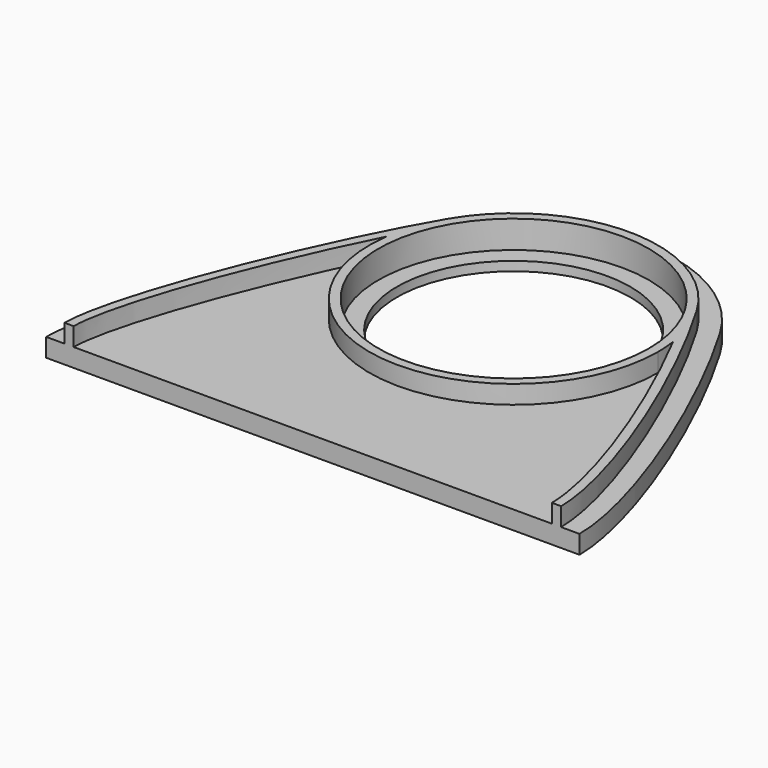
from build123d import *

# Parameters (mm, degrees)
F0_R     = 12.7
F1_DEPTH = 2
F3_DEPTH = 2
F4_DEPTH = 1


# Not quite as in the source:
# - the dataset's text gives a spline's control points without its knots; the knots are read off the source's solid


with BuildPart() as f1:
    # F0 (on Top) → F1 (new body)
    with BuildSketch(Plane.XY):
        with BuildLine():
            add(Edge.make_bspline(
                [(15.2512199078, 66.2827774838), (22.262781729, 54.3783446484), (29, 37.1850712509), (29, 30)],
                knots=[0, 0, 0, 0, 38.8003723689, 38.8003723689, 38.8003723689, 38.8003723689], degree=3))
            ThreePointArc((15.2512199078, 66.2827774838), (0, 75), (-15.2512199078, 66.2827774838))
            add(Edge.make_bspline(
                [(-15.2512199078, 66.2827774838), (-21.2251645455, 56.1400411697), (-29, 37.1850712509), (-29, 30)],
                knots=[0, 0, 0, 0, 38.8003723689, 38.8003723689, 38.8003723689, 38.8003723689], degree=3))
            Line((-29, 30), (-27, 30))
            Line((-27, 30), (27, 30))
            Line((27, 30), (29, 30))
        make_face()
        with Locations((0, 57.3)):
            Circle(F0_R, mode=Mode.SUBTRACT)
    extrude(amount=F1_DEPTH)

    # F2 (on face) → F3 (join)
    with BuildSketch(Plane.XY.offset(2)):
        with BuildLine():
            ThreePointArc((15.5364060101, 59.5605504394), (14.8096872708, 62.5118291359), (13.5279182233, 65.2677743783))
            ThreePointArc((13.5279182233, 65.2677743783), (0, 73), (-13.5279182233, 65.2677743783))
            ThreePointArc((-13.5279182233, 65.2677743783), (-14.8291754406, 62.4561182834), (-15.5529629237, 59.4436754174))
            add(Edge.make_bspline(
                [(-12.666267381, 64.7602728256), (-13.3814975344, 63.5459343458), (-14.3471757573, 61.795170814), (-15.3337673015, 59.8762099433), (-15.5529629237, 59.4436754174)],
                knots=[0, 0, 0, 0, 0.125, 0.160588695, 0.160588695, 0.160588695, 0.160588695], degree=3))
            ThreePointArc((-12.666267381, 64.7602728256), (0, 72), (12.666267381, 64.7602728256))
            add(Edge.make_bspline(
                [(12.666267381, 64.7602728256), (13.6300436519, 63.1239455453), (14.5936812112, 61.3751520533), (15.5364060101, 59.5605504394)],
                knots=[0, 0, 0, 0, 0.1417988525, 0.1417988525, 0.1417988525, 0.1417988525], degree=3))
        make_face()
        with BuildLine():
            ThreePointArc((-15.5529629237, 59.4436754174), (-14.8291754406, 62.4561182834), (-13.5279182233, 65.2677743783))
            add(Edge.make_bspline(
                [(-13.5279182233, 65.2677743783), (-14.2536759146, 64.0355619396), (-15.772450124, 61.2815842663), (-18.1202539958, 56.5478531468), (-20.4180305231, 51.4643495554), (-22.5492955187, 46.2810247995), (-24.3986592394, 41.2483510136), (-25.8510078819, 36.6233031241), (-26.6335925167, 33.3345469461), (-26.9500727399, 31.2110731734), (-27, 30.3588934626), (-27, 30)],
                knots=[0, 0, 0, 0, 0.125, 0.25, 0.375, 0.5, 0.625, 0.75, 0.875, 0.9375, 1, 1, 1, 1], degree=3))
            Line((-27, 30), (-26, 30))
            add(Edge.make_bspline(
                [(-15.5529629237, 59.4436754174), (-16.103659335, 58.3569967289), (-17.432620702, 55.641124998), (-19.4997246297, 51.0680076024), (-21.6176712905, 45.9169669649), (-23.4528661033, 40.9225678129), (-24.6491582432, 37.111718992), (-25.347699755, 34.4173662896), (-25.7291020699, 32.6200108572), (-25.9554408122, 31.0980618143), (-26, 30.3125219854), (-26, 30)],
                knots=[0.160588695, 0.160588695, 0.160588695, 0.160588695, 0.25, 0.375, 0.5, 0.625, 0.75, 0.8125, 0.875, 0.9375, 1, 1, 1, 1], degree=3))
        make_face()
        with BuildLine():
            add(Edge.make_bspline(
                [(13.5279182233, 65.2677743783), (15.2450490143, 62.3523799637), (18.6671458399, 55.8354316971), (22.3671878092, 47.2230529585), (24.6675324684, 40.7998884344), (25.9849445097, 36.4102773166), (26.6779139538, 33.280652434), (26.9557291702, 31.2220902723), (27, 30.3709278734), (27, 30)],
                knots=[0, 0, 0, 0, 0.25, 0.5, 0.625, 0.75, 0.875, 0.9375, 1, 1, 1, 1], degree=3))
            ThreePointArc((13.5279182233, 65.2677743783), (14.8096872708, 62.5118291359), (15.5364060101, 59.5605504394))
            add(Edge.make_bspline(
                [(15.5364060101, 59.5605504394), (16.2557623605, 58.1758990588), (17.7799153794, 55.1090370481), (19.9683054435, 50.2727965075), (22.0085555342, 45.2584906765), (23.7183366896, 40.4837611553), (25.0184785808, 36.1508570007), (25.6948193529, 33.090063524), (25.9598858219, 31.1209960906), (26, 30.3311440115), (26, 30)],
                knots=[0.1417988525, 0.1417988525, 0.1417988525, 0.1417988525, 0.25, 0.375, 0.5, 0.625, 0.75, 0.875, 0.9375, 1, 1, 1, 1], degree=3))
            Line((26, 30), (27, 30))
        make_face()
        with BuildLine():
            ThreePointArc((15.7, 57.3), (15.659048093, 58.4332311418), (15.5364060101, 59.5605504394))
            add(Edge.make_bspline(
                [(12.666267381, 64.7602728256), (13.6300436519, 63.1239455453), (14.5936812112, 61.3751520533), (15.5364060101, 59.5605504394)],
                knots=[0, 0, 0, 0, 0.1417988525, 0.1417988525, 0.1417988525, 0.1417988525], degree=3))
            ThreePointArc((12.666267381, 64.7602728256), (14.1824562489, 61.1662559084), (14.7, 57.3))
            ThreePointArc((14.7, 57.3), (-3.8662559084, 43.1175437511), (-12.666267381, 64.7602728256))
            add(Edge.make_bspline(
                [(-12.666267381, 64.7602728256), (-13.3814975344, 63.5459343458), (-14.3471757573, 61.795170814), (-15.3337673015, 59.8762099433), (-15.5529629237, 59.4436754174)],
                knots=[0, 0, 0, 0, 0.125, 0.160588695, 0.160588695, 0.160588695, 0.160588695], degree=3))
            ThreePointArc((-15.5529629237, 59.4436754174), (-1.0743561091, 41.6368024034), (15.7, 57.3))
        make_face()
    extrude(amount=F3_DEPTH)

    # F4 (cut): a face of the model
    f4_faces = [f1.faces().sort_by_distance(p)[0] for p in [
        (-12.3080112387, 50.0507355546, 2),
    ]]
    extrude(f4_faces, amount=-F4_DEPTH, mode=Mode.SUBTRACT)


solid = f1.part
